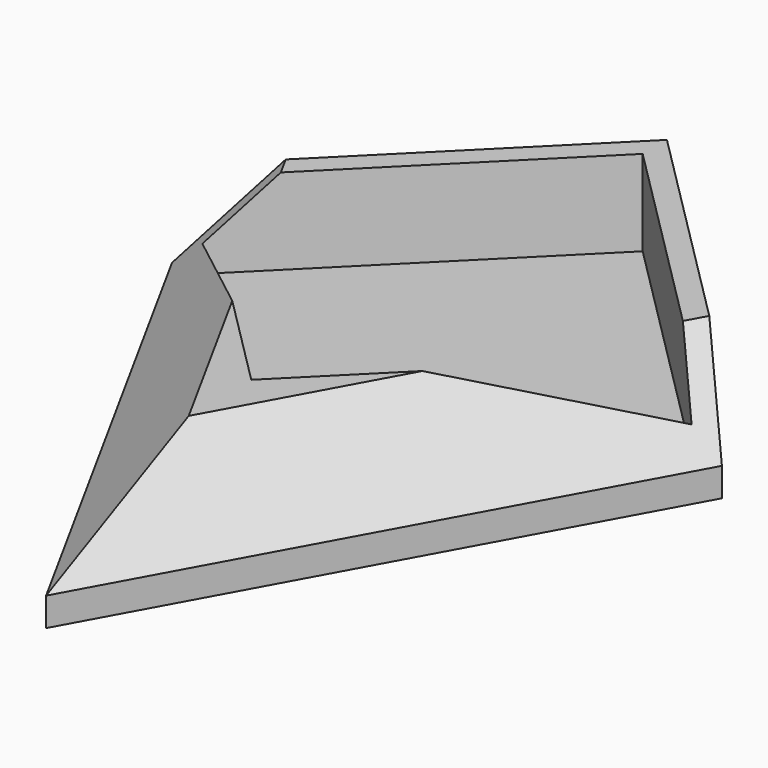
from build123d import *

# Parameters (mm, degrees)
F0_W        = 13.6
F0_H        = 13.6
F1_DEPTH    = 4
F2_W        = 12.1
F2_H        = 12.1
F3_DEPTH    = 3
F5_ANGLE    = 45
F7_DEPTH    = 4
F8_T1_DEPTH = 35.422011596
F8_T3_DEPTH = 35.422011596


# Not quite as in the source:
# - a fillet or chamfer that OpenCascade refuses, or shapes differently, is made with other operations: its cross-section is extruded or revolved along the edge and cut away or added


with BuildPart() as f1:
    # F0 (on Top) → F1 (new body)
    with BuildSketch(Plane.XY):
        Rectangle(F0_W, F0_H)
    extrude(amount=F1_DEPTH)

    # F2 (on face) → F3 (cut)
    with BuildSketch(Plane.XY.offset(4)):
        Rectangle(F2_W, F2_H)
    extrude(amount=-F3_DEPTH, mode=Mode.SUBTRACT)


with BuildPart() as f1_1:
    # F5: moved
    add(f1.part.rotate(Axis((0, 0, 16.5512096137), (0, 0, 1)), F5_ANGLE))

    # F6 (on face) → F7 (join)
    with BuildSketch(Plane(origin=(0, 0, 0), x_dir=(1, 0, 0), z_dir=(0, 0, -1))):
        Polygon((0, 9.6166522241), (9.6166522241, 0), (0, 17.527025193), (-9.6166522241, 0), align=None)
    extrude(amount=-F7_DEPTH)

    # F8: chamfer of 3 on 2 edges, made by hand

    # F8_s2 → F8_t1 (cut)
    with BuildSketch(Plane(origin=(5.9363165934, 10.8193546008, 0), x_dir=(0, 0, 1), z_dir=(-0.4810270984, -0.8767057263, 0))):
        Polygon((4, -5.4309740729), (1, -8.4309740729), (4, -8.4309740729), align=None)
    extrude(amount=F8_T1_DEPTH, mode=Mode.SUBTRACT)

    # F8_s4 → F8_t3 (cut)
    with BuildSketch(Plane(origin=(11.1026308657, -20.2353258031, 0), x_dir=(0, 0, 1), z_dir=(-0.4810270984, 0.8767057263, 0))):
        Polygon((1, -8.4309740729), (4, -5.4309740729), (4, -8.4309740729), align=None)
    extrude(amount=F8_T3_DEPTH, mode=Mode.SUBTRACT)


solid = f1_1.part
